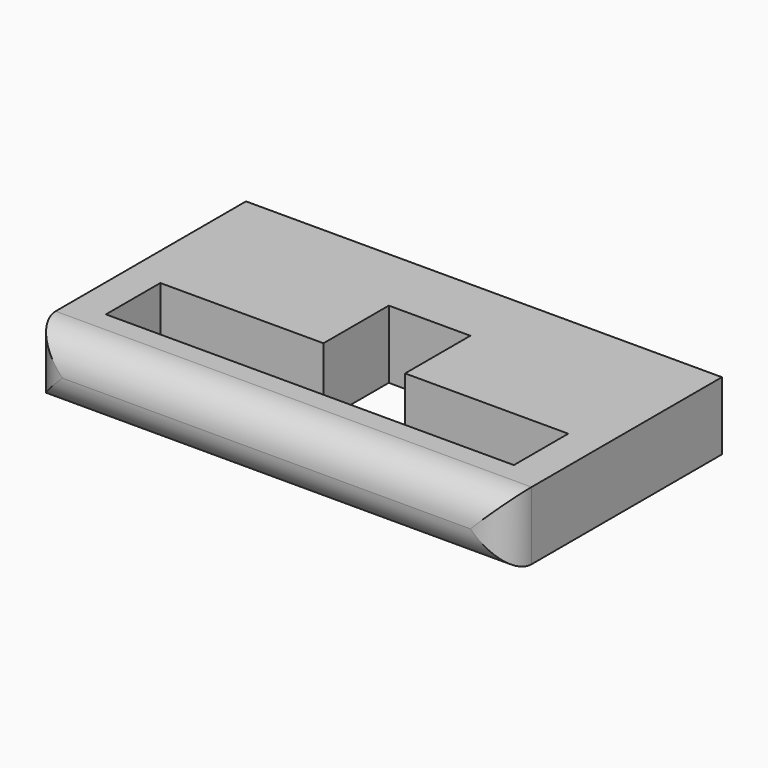
from build123d import *

# Parameters (mm, degrees)
F0_W     = 35
F0_H     = 20
F1_DEPTH = 5
F2_R     = 2.49999


# Not quite as in the source:
# - a fillet or chamfer is up to 0.001 mm smaller than in the source, because OpenCascade refuses the exact size


with BuildPart() as f1:
    # F0 (on Top) → F1 (new body)
    with BuildSketch(Plane.XY):
        Rectangle(F0_W, F0_H)
        Polygon((3, -1), (15, -1), (15, -6), (-15, -6), (-15, -1), (-3, -1), (-3, 5), (3, 5), align=None, mode=Mode.SUBTRACT)
    extrude(amount=F1_DEPTH)

    # F2 (radius 2.5 in the source; OpenCascade refuses exactly that, so slightly less here)
    f2_edges = [f1.edges().sort_by_distance(p)[0] for p in [
        (-17.5, -10, 2.5),
        (17.5, -10, 2.5),
        (0, -10, 0),
        (0, -10, 5),
    ]]
    fillet(f2_edges, radius=F2_R)


solid = f1.part
